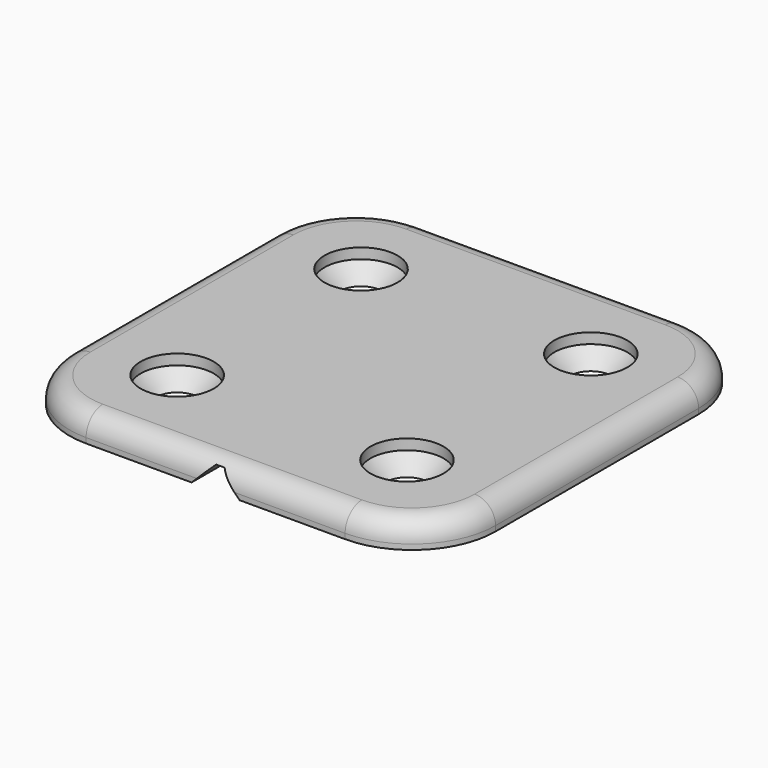
from build123d import *

# Parameters (mm, degrees)
F0_R     = 3.5
F0_R_2   = 2
F1_DEPTH = 1.5
F2_DEPTH = 2.5
F3_R     = 2
F4_SIZE  = 1.49999
F7_DEPTH = 40.301


# Not quite as in the source:
# - a fillet or chamfer is up to 0.001 mm smaller than in the source, because OpenCascade refuses the exact size


with BuildPart() as f1:
    # F0 (on Top) → F1 (new body)
    with BuildSketch(Plane.XY):
        with BuildLine():
            ThreePointArc((20.4, 12.15), (18.0568542495, 17.8068542495), (12.4, 20.15))
            Line((12.4, 20.15), (-12.4, 20.15))
            ThreePointArc((-12.4, 20.15), (-18.0568542495, 17.8068542495), (-20.4, 12.15))
            Line((-20.4, 12.15), (-20.4, -12.15))
            ThreePointArc((-20.4, -12.15), (-18.0568542495, -17.8068542495), (-12.4, -20.15))
            Line((-12.4, -20.15), (12.4, -20.15))
            ThreePointArc((12.4, -20.15), (18.0568542495, -17.8068542495), (20.4, -12.15))
            Line((20.4, -12.15), (20.4, 12.15))
        make_face()
        with Locations((-11, -11)):
            Circle(F0_R, mode=Mode.SUBTRACT)
        with Locations((11, -11)):
            Circle(F0_R, mode=Mode.SUBTRACT)
        with Locations((-11, 11)):
            Circle(F0_R, mode=Mode.SUBTRACT)
        with Locations((11, 11)):
            Circle(F0_R, mode=Mode.SUBTRACT)
        with Locations((-11, 11)):
            Circle(F0_R)
        with Locations((-11, 11)):
            Circle(F0_R_2, mode=Mode.SUBTRACT)
        with Locations((11, 11)):
            Circle(F0_R)
        with Locations((11, 11)):
            Circle(F0_R_2, mode=Mode.SUBTRACT)
        with Locations((11, -11)):
            Circle(F0_R)
        with Locations((11, -11)):
            Circle(F0_R_2, mode=Mode.SUBTRACT)
        with Locations((-11, -11)):
            Circle(F0_R)
        with Locations((-11, -11)):
            Circle(F0_R_2, mode=Mode.SUBTRACT)
    extrude(amount=F1_DEPTH)

    # F0 (on Top) → F2 (join)
    with BuildSketch(Plane.XY):
        with BuildLine():
            ThreePointArc((20.4, 12.15), (18.0568542495, 17.8068542495), (12.4, 20.15))
            Line((12.4, 20.15), (-12.4, 20.15))
            ThreePointArc((-12.4, 20.15), (-18.0568542495, 17.8068542495), (-20.4, 12.15))
            Line((-20.4, 12.15), (-20.4, -12.15))
            ThreePointArc((-20.4, -12.15), (-18.0568542495, -17.8068542495), (-12.4, -20.15))
            Line((-12.4, -20.15), (12.4, -20.15))
            ThreePointArc((12.4, -20.15), (18.0568542495, -17.8068542495), (20.4, -12.15))
            Line((20.4, -12.15), (20.4, 12.15))
        make_face()
        with Locations((-11, -11)):
            Circle(F0_R, mode=Mode.SUBTRACT)
        with Locations((11, -11)):
            Circle(F0_R, mode=Mode.SUBTRACT)
        with Locations((-11, 11)):
            Circle(F0_R, mode=Mode.SUBTRACT)
        with Locations((11, 11)):
            Circle(F0_R, mode=Mode.SUBTRACT)
    extrude(amount=F2_DEPTH)

    # F3
    f3_edges = [f1.edges().sort_by_distance(p)[0] for p in [
        (-18.056854, 17.806854, 2.5),
    ]]
    fillet(f3_edges, radius=F3_R)

    # F4 (size 1.5 in the source; OpenCascade refuses exactly that, so slightly less here)
    f4_edges = [f1.edges().sort_by_distance(p)[0] for p in [
        (-13, 11, 1.5),
        (9, 11, 1.5),
        (9, -11, 1.5),
        (-13, -11, 1.5),
    ]]
    chamfer(f4_edges, length=F4_SIZE)

    # F6 (on offset) → F7 (cut, through all)
    with BuildSketch(Plane.XZ.offset(20.15)):
        Polygon((-0.4, 1.9), (-2.3, 0), (2.3, 0), (0.4, 1.9), align=None)
    extrude(amount=-F7_DEPTH, mode=Mode.SUBTRACT)


solid = f1.part
